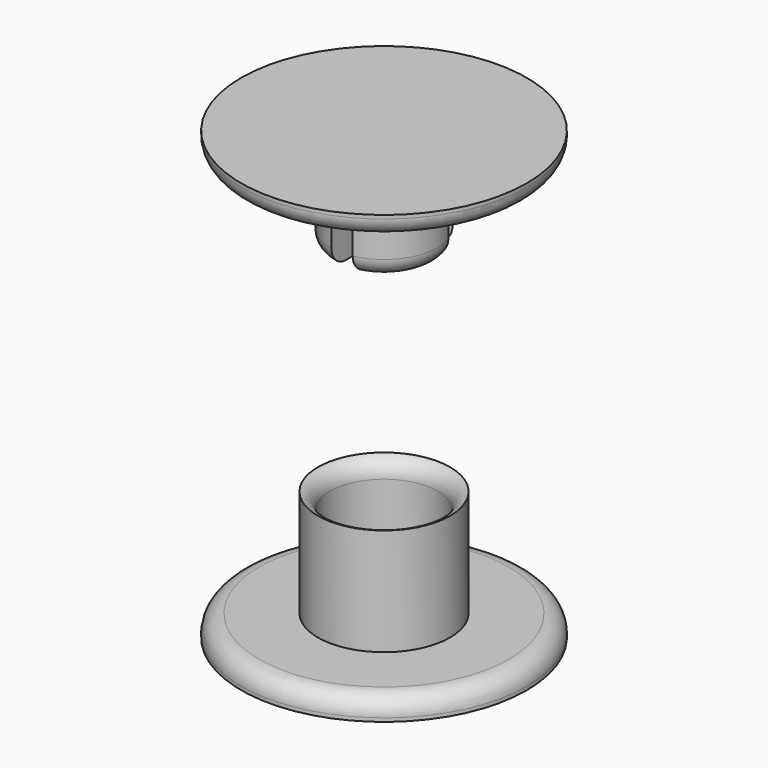
from build123d import *

# Parameters (mm, degrees)
F0_R       = 8
F1_DEPTH   = 1.2
F2_R       = 3.7
F3_DEPTH   = 6
F4_R       = 3
F5_DEPTH   = 5
F7_R       = 8
F8_DEPTH   = 1.2
F9_R       = 3
F10_DEPTH  = 4.6
F11_R      = 0.6
F12_DEPTH  = 4
F13_2_F1_R = 1
F13_2_F2_R = 1
F13_2_F3_R = 1
F13_2_F4_R = 1


# Not quite as in the source:
# - a fillet or chamfer that OpenCascade refuses, or shapes differently, is made with other operations: its cross-section is extruded or revolved along the edge and cut away or added
# - a feature names something its author has since deleted; it is built from what else it names


with BuildPart() as f1:
    # F0 (on Top) → F1 (new body)
    with BuildSketch(Plane.XY):
        Circle(F0_R)
    extrude(amount=F1_DEPTH)

    # F2 (on face) → F3 (join)
    with BuildSketch(Plane.XY.offset(1.2)):
        Circle(F2_R)
    extrude(amount=F3_DEPTH)

    # F4 (on face) → F5 (cut)
    with BuildSketch(Plane.XY.offset(7.2)):
        Circle(F4_R)
    extrude(amount=-F5_DEPTH, mode=Mode.SUBTRACT)

    # F13: fillet of radius 1 on 2 edges, made by hand

    # F13_s1 → F13_t2 (revolve, cut)
    with BuildSketch(Plane.XZ):
        with BuildLine():
            ThreePointArc((3.7, 7.2), (3.1937742252, 6.8376687769), (3, 6.2460607986))
            Line((3, 6.2460607986), (3, 7.2))
            Line((3, 7.2), (3.7, 7.2))
        make_face()
    revolve(axis=Axis((0, 0, 7.2), (0, 0, 1)), mode=Mode.SUBTRACT)

    # F13_s3 → F13_t4 (revolve, cut)
    with BuildSketch(Plane.XZ):
        with BuildLine():
            ThreePointArc((8, 0.2), (7.7071067812, 0.9071067812), (7, 1.2))
            Line((7, 1.2), (8, 1.2))
            Line((8, 1.2), (8, 0.2))
        make_face()
    revolve(axis=Axis((0, 0, 1.2), (0, 0, 1)), mode=Mode.SUBTRACT)


with BuildPart() as f8:
    # F7 (on offset) → F8 (new body)
    with BuildSketch(Plane.XY.offset(25)):
        Circle(F7_R)
    extrude(amount=-F8_DEPTH)

    # F9 (on face) → F10 (join)
    with BuildSketch(Plane(origin=(0, 0, 23.8), x_dir=(1, 0, 0), z_dir=(0, 0, -1))):
        Circle(F9_R)
    extrude(amount=F10_DEPTH)

    # F11 (on face) → F12 (cut)
    with BuildSketch(Plane(origin=(0, 0, 19.2), x_dir=(1, 0, 0), z_dir=(0, 0, -1))):
        with BuildLine():
            Line((2.8455844123, -0.9500786034), (0.6, 0.3464101615))
            Line((0.6, 0.3464101615), (0.6, 2.9393876913))
            ThreePointArc((0.6, 2.9393876913), (0, 3), (-0.6, 2.9393876913))
            Line((-0.6, 2.9393876913), (-0.6, 0.3464101615))
            Line((-0.6, 0.3464101615), (-2.8455844123, -0.9500786034))
            ThreePointArc((-2.8455844123, -0.9500786034), (-2.5980762114, -1.5), (-2.2455844123, -1.9893090879))
            Line((-2.2455844123, -1.9893090879), (0, -0.692820323))
            Line((0, -0.692820323), (2.2455844123, -1.9893090879))
            ThreePointArc((2.2455844123, -1.9893090879), (2.5980762114, -1.5), (2.8455844123, -0.9500786034))
        make_face()
        Circle(F11_R, mode=Mode.SUBTRACT)
        Circle(F11_R)
    extrude(amount=-F12_DEPTH, mode=Mode.SUBTRACT)

    # F13#2: fillet of radius 1 on 5 edges, made by hand

    # F13_2_f1
    f13_2_f1_edges = [f8.edges().sort_by_distance(p)[0] for p in [
        (-8, 0, 23.8),
    ]]
    fillet(f13_2_f1_edges, radius=F13_2_F1_R)

    # F13_2_f2
    f13_2_f2_edges = [f8.edges().sort_by_distance(p)[0] for p in [
        (2.9611444778, 0.4812726687, 19.2),
        (2.3237900077, -1.8973665961, 19.2),
    ]]
    fillet(f13_2_f2_edges, radius=F13_2_F2_R)

    # F13_2_f3
    f13_2_f3_edges = [f8.edges().sort_by_distance(p)[0] for p in [
        (0, 3, 19.2),
    ]]
    fillet(f13_2_f3_edges, radius=F13_2_F3_R)

    # F13_2_f4
    f13_2_f4_edges = [f8.edges().sort_by_distance(p)[0] for p in [
        (-2.5980762114, -1.5, 19.2),
    ]]
    fillet(f13_2_f4_edges, radius=F13_2_F4_R)


solid = Compound([f1.part, f8.part])
